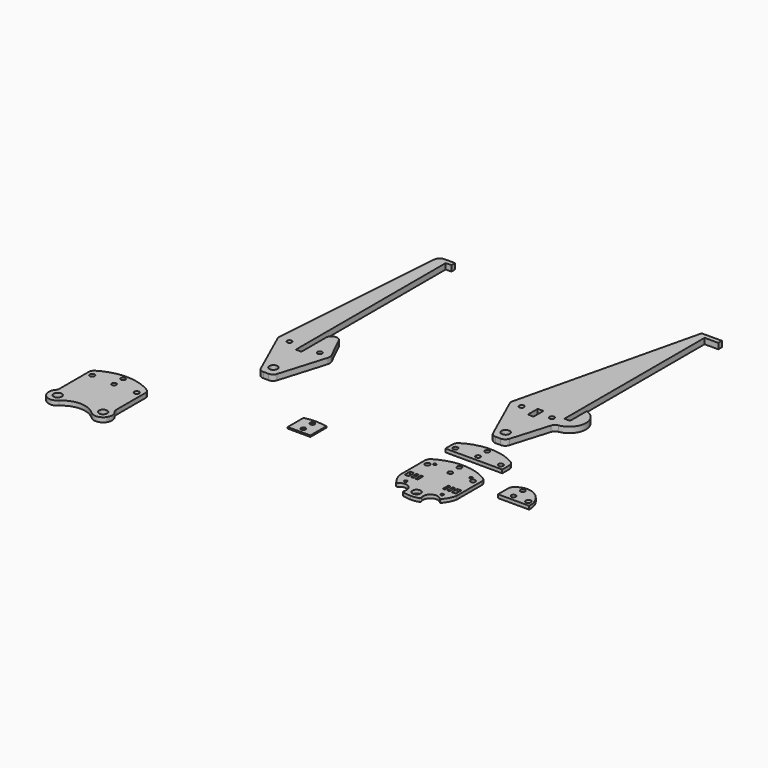
from build123d import *

# Parameters (mm, degrees)
F0_R      = 1.25
F0_W      = 3.5
F0_H      = 6
F0_W_2    = 2
F0_R_2    = 3.555
F0_R_3    = 2.1
F0_R_4    = 2
F1_DEPTH  = 3
F2_DEPTH  = 3
F4_R      = 2.1
F4_R_2    = 2.25
F5_DEPTH  = 25
F6_DEPTH  = 3
F8_DEPTH  = 1.25
F0_R_5    = 3.6
F9_DEPTH  = 5
F0_W_3    = 5
F0_H_2    = 10.7942670584
F10_DEPTH = 4


# Not quite as in the source:
# - a feature names something its author has since deleted; it is built from what else it names


with BuildPart() as f1:
    # F0 (on Top) → F1 (new body)
    with BuildSketch(Plane.XY):
        with BuildLine():
            Line((25, 14.3136761677), (-25, 14.3136761677))
            Line((-25, 14.3136761677), (-25, -5.6028405869))
            ThreePointArc((-25, -5.6028405869), (-23.0117824833, -10.8325706042), (-19.9442440013, -15.5115974911))
            ThreePointArc((-19.9442440013, -15.5115974911), (-19.2052482882, -15.8754446325), (-18.443850882, -15.5611622815))
            ThreePointArc((-18.443850882, -15.5611622815), (-10.1760612052, -14.5858281895), (-7.7862204272, -22.5605560084))
            ThreePointArc((-7.7862204272, -22.5605560084), (-7.7721201862, -23.38414607), (-7.1446119827, -23.9177497252))
            ThreePointArc((-7.1446119827, -23.9177497252), (-3.6076561704, -24.6722072912), (0, -24.9253467642))
            ThreePointArc((0, -24.9253467642), (3.6076561704, -24.6722072912), (7.1446119827, -23.9177497252))
            ThreePointArc((7.1446119827, -23.9177497252), (7.7721201862, -23.38414607), (7.7862204272, -22.5605560084))
            ThreePointArc((7.7862204272, -22.5605560084), (10.1760612052, -14.5858281895), (18.443850882, -15.5611622815))
            ThreePointArc((18.443850882, -15.5611622815), (19.2052482882, -15.8754446325), (19.9442440013, -15.5115974911))
            ThreePointArc((19.9442440013, -15.5115974911), (23.0117824833, -10.8325706042), (25, -5.6028405869))
            Line((25, -5.6028405869), (25, 14.3136761677))
        make_face()
        with Locations((-16, -10)):
            Circle(F0_R, mode=Mode.SUBTRACT)
        with Locations((-20.75, 0)):
            Rectangle(F0_W, F0_H, mode=Mode.SUBTRACT)
        with Locations((-16, 0)):
            Rectangle(F0_W_2, F0_H, mode=Mode.SUBTRACT)
        with Locations((-12, 0)):
            Rectangle(F0_W_2, F0_H, mode=Mode.SUBTRACT)
        with Locations((0, -18)):
            Circle(F0_R_2, mode=Mode.SUBTRACT)
        with Locations((16, -10)):
            Circle(F0_R, mode=Mode.SUBTRACT)
        with Locations((12, 0)):
            Rectangle(F0_W_2, F0_H, mode=Mode.SUBTRACT)
        with Locations((16, 0)):
            Rectangle(F0_W_2, F0_H, mode=Mode.SUBTRACT)
        with Locations((20.75, 0)):
            Rectangle(F0_W, F0_H, mode=Mode.SUBTRACT)
        with BuildLine():
            ThreePointArc((-22.6164226719, 26.5744662824), (-24.3636059263, 24.7547708647), (-25, 22.3136761677))
            Line((-25, 22.3136761677), (-25, 14.3136761677))
            Line((-25, 14.3136761677), (25, 14.3136761677))
            Line((25, 14.3136761677), (25, 22.3136761677))
            ThreePointArc((25, 22.3136761677), (24.3636059263, 24.7547708647), (22.6164226719, 26.5744662824))
            ThreePointArc((22.6164226719, 26.5744662824), (0, 32.964214922), (-22.6164226719, 26.5744662824))
        make_face()
        with Locations((-20, 19)):
            Circle(F0_R_3, mode=Mode.SUBTRACT)
        with Locations((0, 19)):
            Circle(F0_R_4, mode=Mode.SUBTRACT)
        with Locations((20, 19)):
            Circle(F0_R_3, mode=Mode.SUBTRACT)
        with Locations((-16, 22)):
            Circle(F0_R, mode=Mode.SUBTRACT)
        with Locations((0, 29)):
            Circle(F0_R_4, mode=Mode.SUBTRACT)
        with Locations((16, 22)):
            Circle(F0_R, mode=Mode.SUBTRACT)
    extrude(amount=F1_DEPTH)


with BuildPart() as f2:
    # F0 (on Top) → F2 (new body)
    with BuildSketch(Plane.XY):
        with BuildLine():
            ThreePointArc((-22.6164226719, 26.5744662824), (-24.3636059263, 24.7547708647), (-25, 22.3136761677))
            Line((-25, 22.3136761677), (-25, 14.3136761677))
            Line((-25, 14.3136761677), (25, 14.3136761677))
            Line((25, 14.3136761677), (25, 22.3136761677))
            ThreePointArc((25, 22.3136761677), (24.3636059263, 24.7547708647), (22.6164226719, 26.5744662824))
            ThreePointArc((22.6164226719, 26.5744662824), (0, 32.964214922), (-22.6164226719, 26.5744662824))
        make_face()
        with Locations((-20, 19)):
            Circle(F0_R_3, mode=Mode.SUBTRACT)
        with Locations((0, 19)):
            Circle(F0_R_4, mode=Mode.SUBTRACT)
        with Locations((20, 19)):
            Circle(F0_R_3, mode=Mode.SUBTRACT)
        with Locations((-16, 22)):
            Circle(F0_R, mode=Mode.SUBTRACT)
        with Locations((0, 29)):
            Circle(F0_R_4, mode=Mode.SUBTRACT)
        with Locations((16, 22)):
            Circle(F0_R, mode=Mode.SUBTRACT)
        with Locations((-16, 22)):
            Circle(F0_R)
        with Locations((16, 22)):
            Circle(F0_R)
    extrude(amount=F2_DEPTH)


with BuildPart() as f2_1:
    # F3: moved
    add(f2.part.moved(Location((55.75, 0, 0))))

    # F4 (on face) → F5 (cut)
    with BuildSketch(Plane.XY.offset(3)):
        with BuildLine():
            Line((30.75, 14.3136761677), (45.75, 14.3136761677))
            Line((45.75, 14.3136761677), (45.75, 25.7562933257))
            ThreePointArc((45.75, 25.7562933257), (46.2050390496, 27.8403590538), (47.4873319836, 29.5450922667))
            ThreePointArc((47.4873319836, 29.5450922667), (51.3440284338, 31.9183440188), (55.75, 32.964214922))
            ThreePointArc((55.75, 32.964214922), (43.9991334133, 31.3361124445), (33.1335773281, 26.5744662824))
            ThreePointArc((33.1335773281, 26.5744662824), (31.3863940737, 24.7547708647), (30.75, 22.3136761677))
            Line((30.75, 22.3136761677), (30.75, 14.3136761677))
        make_face()
        with Locations((35.75, 19)):
            Circle(F4_R, mode=Mode.SUBTRACT)
        with Locations((42.75, 19)):
            Circle(F4_R_2, mode=Mode.SUBTRACT)
        with BuildLine():
            ThreePointArc((58.8838195988, 32.8504511649), (60.9470746388, 32.3880346997), (62.9193889887, 31.6259149894))
            ThreePointArc((62.9193889887, 31.6259149894), (70.6461883393, 24.5054009937), (73.2023363863, 14.3136761677))
            Line((73.2023363863, 14.3136761677), (80.75, 14.3136761677))
            Line((80.75, 14.3136761677), (80.75, 22.3136761677))
            ThreePointArc((80.75, 22.3136761677), (80.1136059263, 24.7547708647), (78.3664226719, 26.5744662824))
            ThreePointArc((78.3664226719, 26.5744662824), (69.0020089349, 30.8824353153), (58.8838195988, 32.8504511649))
        make_face()
        with Locations((75.75, 19)):
            Circle(F4_R, mode=Mode.SUBTRACT)
        with Locations((42.75, 19)):
            Circle(F4_R_2)
        with Locations((68.75, 19)):
            Circle(F4_R_2)
    extrude(amount=-F5_DEPTH, mode=Mode.SUBTRACT)


with BuildPart() as f6:
    # F0 (on Top) → F6 (new body)
    with BuildSketch(Plane.XY):
        with BuildLine():
            ThreePointArc((-22.6164226719, 26.5744662824), (-24.3636059263, 24.7547708647), (-25, 22.3136761677))
            Line((-25, 22.3136761677), (-25, 14.3136761677))
            Line((-25, 14.3136761677), (25, 14.3136761677))
            Line((25, 14.3136761677), (25, 22.3136761677))
            ThreePointArc((25, 22.3136761677), (24.3636059263, 24.7547708647), (22.6164226719, 26.5744662824))
            ThreePointArc((22.6164226719, 26.5744662824), (0, 32.964214922), (-22.6164226719, 26.5744662824))
        make_face()
        with Locations((-20, 19)):
            Circle(F0_R_3, mode=Mode.SUBTRACT)
        with Locations((0, 19)):
            Circle(F0_R_4, mode=Mode.SUBTRACT)
        with Locations((20, 19)):
            Circle(F0_R_3, mode=Mode.SUBTRACT)
        with Locations((-16, 22)):
            Circle(F0_R, mode=Mode.SUBTRACT)
        with Locations((0, 29)):
            Circle(F0_R_4, mode=Mode.SUBTRACT)
        with Locations((16, 22)):
            Circle(F0_R, mode=Mode.SUBTRACT)
        with Locations((16, 22)):
            Circle(F0_R)
        with Locations((-16, 22)):
            Circle(F0_R)
    extrude(amount=F6_DEPTH)


with BuildPart() as f6_1:
    # F7: moved
    add(f6.part.moved(Location((0, 30.6, 0))))


with BuildPart() as f8:
    # F0 (on Top) → F8 (new body)
    with BuildSketch(Plane.XY):
        with BuildLine():
            Line((-111.7582723053, 4.8228372639), (-111.7582723053, 22.3005958048))
            ThreePointArc((-111.7582723053, 22.3005958048), (-121.7582723053, 23.4733760182), (-131.7582723053, 22.3005958048))
            Line((-131.7582723053, 22.3005958048), (-131.7582723053, 4.8228372639))
            Line((-131.7582723053, 4.8228372639), (-111.7582723053, 4.8228372639))
        make_face()
        with Locations((-121.7352634446, 9.5091610962)):
            Circle(F0_R_4, mode=Mode.SUBTRACT)
        with Locations((-121.7582723053, 19.5091610962)):
            Circle(F0_R_4, mode=Mode.SUBTRACT)
    extrude(amount=F8_DEPTH)


with BuildPart() as f9:
    # F0 (on Top) → F9 (new body)
    with BuildSketch(Plane.XY):
        with BuildLine():
            Line((-194.8590046924, 92.5738288486), (-194.8590046924, 103.368095907))
            Line((-194.8590046924, 103.368095907), (-194.8590046924, 257.5738288486))
            Line((-194.8590046924, 257.5738288486), (-189.8590046924, 257.5738288486))
            Line((-189.8590046924, 257.5738288486), (-189.8590046924, 261.5738288486))
            Line((-189.8590046924, 261.5738288486), (-194.8590046924, 261.5738288486))
            Line((-194.8590046924, 261.5738288486), (-199.3433624056, 261.5738288486))
            ThreePointArc((-199.3433624056, 261.5738288486), (-202.7494446266, 260.2342391951), (-204.3304258465, 256.9332704103))
            Line((-204.3304258465, 256.9332704103), (-215.6025990743, 100.5377697483))
            ThreePointArc((-215.6025990743, 100.5377697483), (-215.5391291879, 99.3075661588), (-215.1768110972, 98.1302153619))
            Line((-215.1768110972, 98.1302153619), (-196.1844668419, 55.8330758659))
            ThreePointArc((-196.1844668419, 55.8330758659), (-194.3397550048, 53.6835367206), (-191.623191378, 52.8811886907))
            Line((-191.623191378, 52.8811886907), (-190.2272651168, 52.8811886907))
            Line((-190.2272651168, 52.8811886907), (-187.0122555796, 52.8811886907))
            ThreePointArc((-187.0122555796, 52.8811886907), (-184.0285668791, 53.8690070224), (-182.2238151365, 56.4421479951))
            Line((-182.2238151365, 56.4421479951), (-170.0274270321, 97.0259051049))
            ThreePointArc((-170.0274270321, 97.0259051049), (-169.7936886967, 99.2438672192), (-170.3861668977, 101.3939739912))
            Line((-170.3861668977, 101.3939739912), (-180.3695141374, 121.757355578))
            ThreePointArc((-180.3695141374, 121.757355578), (-185.9887274958, 124.427039679), (-189.8590046924, 119.5563388683))
            Line((-189.8590046924, 119.5563388683), (-189.8590046924, 103.368095907))
            Line((-189.8590046924, 103.368095907), (-189.8590046924, 92.5738288486))
            Line((-189.8590046924, 92.5738288486), (-194.8590046924, 92.5738288486))
        make_face()
        with Locations((-190.2272651168, 62.2803126574)):
            Circle(F0_R_5, mode=Mode.SUBTRACT)
        with Locations((-205.6932300329, 99.2803126574)):
            Circle(F0_R_3, mode=Mode.SUBTRACT)
        with Locations((-179.0247793518, 99.2803126574)):
            Circle(F0_R_3, mode=Mode.SUBTRACT)
    extrude(amount=F9_DEPTH)


with BuildPart() as f9b:
    # F0 (on Top) → F9, piece 2 (new body)
    with BuildSketch(Plane.XY):
        with BuildLine():
            Line((18.5583842257, 127.613979894), (13.5583842257, 127.613979894))
            Line((13.5583842257, 127.613979894), (13.5583842257, 281.8197128356))
            Line((13.5583842257, 281.8197128356), (25.6206393242, 281.8197128356))
            Line((25.6206393242, 281.8197128356), (25.6206393242, 285.8197128356))
            Line((25.6206393242, 285.8197128356), (13.5583842257, 285.8197128356))
            Line((13.5583842257, 285.8197128356), (7.8031995196, 285.8197128356))
            Line((7.8031995196, 285.8197128356), (-30.6902153493, 124.7836537353))
            ThreePointArc((-30.6902153493, 124.7836537353), (-30.6267454629, 123.5534501458), (-30.2644273722, 122.3760993489))
            Line((-30.2644273722, 122.3760993489), (-11.2720831169, 80.0789598529))
            ThreePointArc((-11.2720831169, 80.0789598529), (-9.4273712798, 77.9294207076), (-6.710807653, 77.1270726777))
            Line((-6.710807653, 77.1270726777), (-5.3148813918, 77.1270726777))
            Line((-5.3148813918, 77.1270726777), (-2.0998718546, 77.1270726777))
            ThreePointArc((-2.0998718546, 77.1270726777), (0.8838168459, 78.1148910094), (2.6885685885, 80.6880319821))
            Line((2.6885685885, 80.6880319821), (12.6697822619, 113.9007460998))
            ThreePointArc((12.6697822619, 113.9007460998), (14.1786026544, 116.2358400499), (16.7013769772, 117.4040919274))
            ThreePointArc((16.7013769772, 117.4040919274), (29.1226354183, 130.9574152191), (18.5583842257, 146.003239565))
            Line((18.5583842257, 146.003239565), (18.5583842257, 127.613979894))
        make_face()
        with Locations((-5.3148813918, 86.5261966444)):
            Circle(F0_R_5, mode=Mode.SUBTRACT)
        with Locations((-20.7808463079, 123.5261966444)):
            Circle(F0_R_3, mode=Mode.SUBTRACT)
        with Locations((-7.4466209674, 122.2168463648)):
            Rectangle(F0_W_3, F0_H_2, mode=Mode.SUBTRACT)
        with Locations((5.8876043732, 123.5261966444)):
            Circle(F0_R_3, mode=Mode.SUBTRACT)
    extrude(amount=F9_DEPTH)


with BuildPart() as f10:
    # F0 (on Top) → F10 (new body)
    with BuildSketch(Plane.XY):
        with BuildLine():
            Line((-236.4682501332, -26.4339604817), (-236.4682501332, -20.7362178037))
            ThreePointArc((-236.4682501332, -20.7362178037), (-236.629963782, -19.4748751919), (-237.1046442069, -18.2951231066))
            ThreePointArc((-237.1046442069, -18.2951231066), (-237.8615864864, -17.2732743536), (-238.8518274612, -16.475427689))
            ThreePointArc((-238.8518274612, -16.475427689), (-261.4682501332, -10.0856790494), (-284.0846728051, -16.475427689))
            ThreePointArc((-284.0846728051, -16.475427689), (-285.07491378, -17.2732743536), (-285.8318560594, -18.2951231066))
            ThreePointArc((-285.8318560594, -18.2951231066), (-286.3065364843, -19.4748751919), (-286.4682501332, -20.7362178037))
            Line((-286.4682501332, -20.7362178037), (-286.4682501332, -26.4339604817))
            Line((-286.4682501332, -26.4339604817), (-286.4682501332, -52.7914252395))
            ThreePointArc((-286.4682501332, -52.7914252395), (-286.7631297332, -54.4831232096), (-287.6129869419, -55.9752822913))
            ThreePointArc((-287.6129869419, -55.9752822913), (-289.3215119859, -59.6949945566), (-288.9581588596, -63.7721616698))
            ThreePointArc((-288.9581588596, -63.7721616698), (-288.6115256219, -64.5047812938), (-288.2524077082, -65.2313626307))
            ThreePointArc((-288.2524077082, -65.2313626307), (-282.4298412114, -68.9609505854), (-275.8833560228, -66.7348242196))
            ThreePointArc((-275.8833560228, -66.7348242196), (-261.4682501332, -61.0606680742), (-247.0531442436, -66.7348242196))
            ThreePointArc((-247.0531442436, -66.7348242196), (-240.5066590549, -68.9609505854), (-234.6840925581, -65.2313626307))
            ThreePointArc((-234.6840925581, -65.2313626307), (-234.3249746444, -64.5047812938), (-233.9783414067, -63.7721616698))
            ThreePointArc((-233.9783414067, -63.7721616698), (-233.6149882804, -59.6949945566), (-235.3235133244, -55.9752822913))
            ThreePointArc((-235.3235133244, -55.9752822913), (-236.1733705331, -54.4831232096), (-236.4682501332, -52.7914252395))
            Line((-236.4682501332, -52.7914252395), (-236.4682501332, -26.4339604817))
        make_face()
        with Locations((-281.4682501332, -61.0498939714)):
            Circle(F0_R_2, mode=Mode.SUBTRACT)
        with BuildLine():
            ThreePointArc((-284.1558727434, -46.4932054196), (-281.3683666251, -38.0794065672), (-284.9856109262, -29.9875745648))
            ThreePointArc((-284.9856109262, -29.9875745648), (-279.4695178628, -42.7891726866), (-286.4682501332, -54.8442937464))
            ThreePointArc((-286.4682501332, -54.8442937464), (-285.2592166315, -53.0093252228), (-285.1687411949, -50.8137192275))
            ThreePointArc((-285.1687411949, -50.8137192275), (-285.1678840433, -48.5349386731), (-284.1558727434, -46.4932054196))
        make_face(mode=Mode.SUBTRACT)
        with Locations((-241.4682501332, -61.0498939714)):
            Circle(F0_R_2, mode=Mode.SUBTRACT)
        with BuildLine():
            ThreePointArc((-236.4682501332, -54.8442937464), (-243.4669824035, -42.7891726866), (-237.9508893401, -29.9875745648))
            ThreePointArc((-237.9508893401, -29.9875745648), (-241.5681336413, -38.0794065672), (-238.7806275229, -46.4932054196))
            ThreePointArc((-238.7806275229, -46.4932054196), (-237.768616223, -48.5349386731), (-237.7677590714, -50.8137192275))
            ThreePointArc((-237.7677590714, -50.8137192275), (-237.6772836349, -53.0093252228), (-236.4682501332, -54.8442937464))
        make_face(mode=Mode.SUBTRACT)
        with Locations((-281.4682501332, -23.0498939714)):
            Circle(F0_R_3, mode=Mode.SUBTRACT)
        with Locations((-261.4682501332, -24.0498939714)):
            Circle(F0_R_4, mode=Mode.SUBTRACT)
        with Locations((-261.4682501332, -14.0498939714)):
            Circle(F0_R_4, mode=Mode.SUBTRACT)
        with Locations((-241.4682501332, -24.0498939714)):
            Circle(F0_R_3, mode=Mode.SUBTRACT)
        with BuildLine():
            ThreePointArc((-286.4682501332, -54.8442937464), (-279.4695178628, -42.7891726866), (-284.9856109262, -29.9875745648))
            ThreePointArc((-284.9856109262, -29.9875745648), (-281.3683666251, -38.0794065672), (-284.1558727434, -46.4932054196))
            ThreePointArc((-284.1558727434, -46.4932054196), (-285.1678840433, -48.5349386731), (-285.1687411949, -50.8137192275))
            ThreePointArc((-285.1687411949, -50.8137192275), (-285.2592166315, -53.0093252228), (-286.4682501332, -54.8442937464))
        make_face()
        with BuildLine():
            ThreePointArc((-238.7806275229, -46.4932054196), (-241.5681336413, -38.0794065672), (-237.9508893401, -29.9875745648))
            ThreePointArc((-237.9508893401, -29.9875745648), (-243.4669824035, -42.7891726866), (-236.4682501332, -54.8442937464))
            ThreePointArc((-236.4682501332, -54.8442937464), (-237.6772836349, -53.0093252228), (-237.7677590714, -50.8137192275))
            ThreePointArc((-237.7677590714, -50.8137192275), (-237.768616223, -48.5349386731), (-238.7806275229, -46.4932054196))
        make_face()
    extrude(amount=F10_DEPTH)


solid = Compound([f1.part, f2_1.part, f6_1.part, f8.part, f9.part, f9b.part, f10.part])
